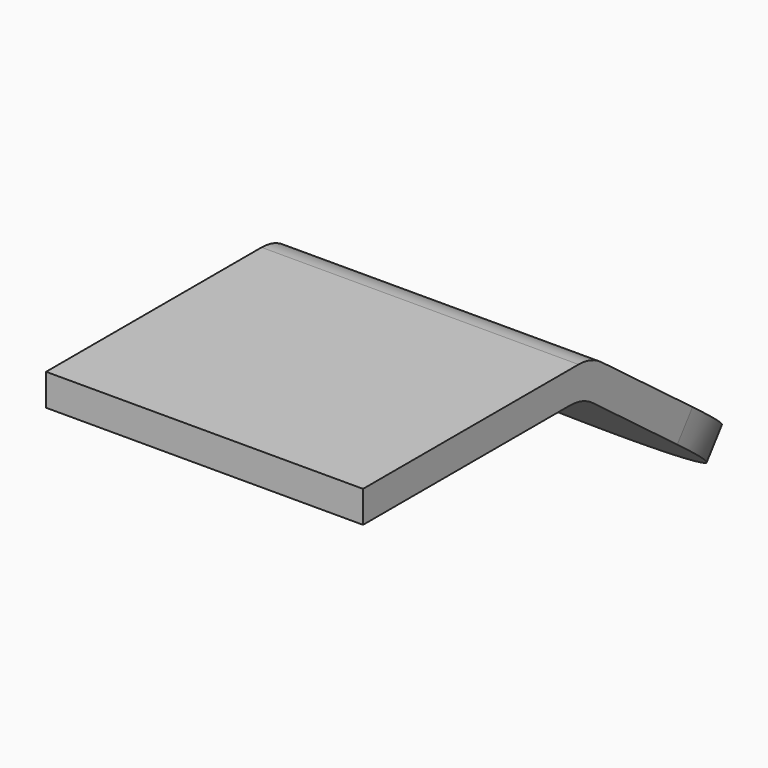
from build123d import *

# Parameters (mm, degrees)
F1_DEPTH = 10
F3_D     = 3.3
F4_R     = 3
F5_R     = 9.99999


# Not quite as in the source:
# - a fillet or chamfer is up to 0.001 mm smaller than in the source, because OpenCascade refuses the exact size


with BuildPart() as f1:
    # F0 (on Right) → F1 (new body, symmetric)
    with BuildSketch(Plane.YZ):
        Polygon((-8.9946911595, 33.2547011177), (-26.9946911595, 33.2547011177), (-26.9946911595, 31.2547011177), (-9.6638817985, 31.2547011177), (5.7743889952, 19.6211296345), (6.9780190415, 21.2184006546), align=None)
    extrude(amount=F1_DEPTH, both=True)

    # F3 (through all)
    with Locations(Plane(origin=(0, 12.7255260612, 16.8873434619), x_dir=(1, 0, 0), z_dir=(0, 0.6018150232, 0.79863551))):
        with Locations((0, -17.1966584849)):
            Hole(F3_D / 2)

    # F4
    f4_edges = [f1.edges().sort_by_distance(p)[0] for p in [
        (0, -8.994691, 33.254701),
        (0, -9.663882, 31.254701),
    ]]
    fillet(f4_edges, radius=F4_R)

    # F5 (radius 10 in the source; OpenCascade refuses exactly that, so slightly less here)
    f5_edges = [f1.edges().sort_by_distance(p)[0] for p in [
        (10, 6.376204, 20.419765),
        (-10, 6.376204, 20.419765),
    ]]
    fillet(f5_edges, radius=F5_R)


solid = f1.part
